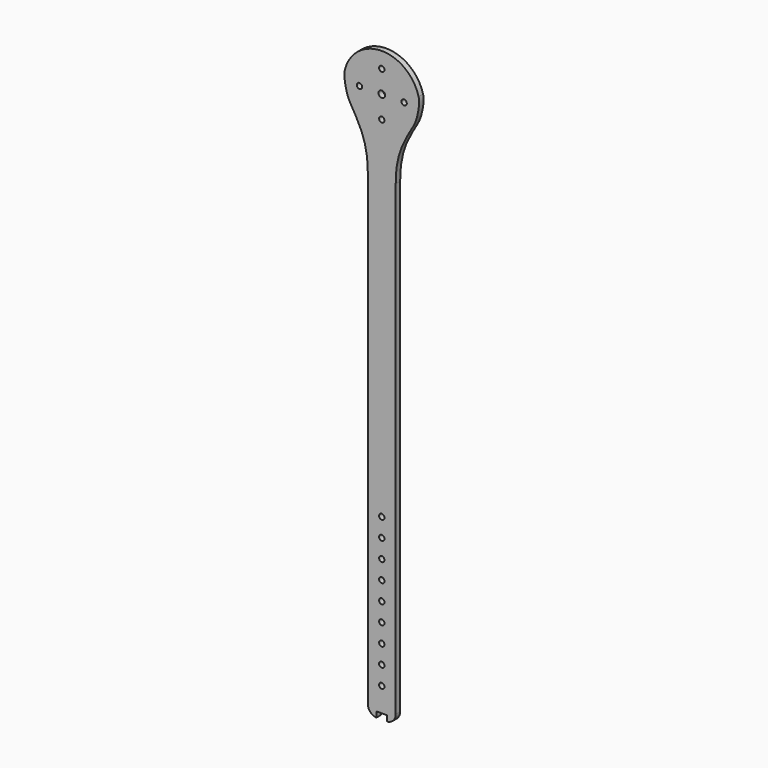
from build123d import *

# Parameters (mm, degrees)
F1_DEPTH        = 3
F2_R            = 1.7859375
F3_DEPTH        = 25
F4_T1_DEPTH     = 27.9314560345
F6_R            = 1.45
F7_DEPTH        = 25
F7_COPIES_COUNT = 4
F8_R            = 1.45
F9_DEPTH        = 25


# Not quite as in the source:
# - a fillet or chamfer that OpenCascade refuses, or shapes differently, is made with other operations: its cross-section is extruded or revolved along the edge and cut away or added
# - a pattern or mirror of a feature is missing from the dataset's text; its kind, count and spacing are read off the source's solid


with BuildPart() as f1:
    # F0 (on Front) → F1 (new body)
    with BuildSketch(Plane.XZ):
        with BuildLine():
            ThreePointArc((-17.7535207776, 10.25), (-18.9395304165, 7.8450103635), (-19.8014794389, 5.3057904246))
            add(Edge.make_bspline(
                [(-19.8014794389, 5.3057904246), (-20.454122155, 2.8700946489), (-19.9763700286, -0.7893865531), (-18.8355536126, -5.0469713795)],
                knots=[0, 0, 0, 0, 10.3977252163, 10.3977252163, 10.3977252163, 10.3977252163], degree=3))
            ThreePointArc((-18.8355536126, -5.0469713795), (-19.3331747968, 2.5452607483), (-16.8874953738, 9.75))
            Line((-16.8874953738, 9.75), (-17.7535207776, 10.25))
        make_face()
        with BuildLine():
            add(Edge.make_bspline(
                [(19.8014794389, 5.3057904246), (20.454122155, 2.8700946489), (19.9763700286, -0.7893865531), (18.8355536126, -5.0469713795)],
                knots=[0, 0, 0, 0, 10.3977252163, 10.3977252163, 10.3977252163, 10.3977252163], degree=3))
            ThreePointArc((19.8014794389, 5.3057904246), (2.6757869405, 20.3246196582), (-17.7535207776, 10.25))
            Line((-17.7535207776, 10.25), (-16.8874953738, 9.75))
            ThreePointArc((-16.8874953738, 9.75), (5.0469713795, 18.8355536126), (19.5, 0))
            ThreePointArc((19.5, 0), (19.3331747968, -2.5452607483), (18.8355536126, -5.0469713795))
        make_face()
        with BuildLine():
            ThreePointArc((-18.8355536126, -5.0469713795), (-18.015650884, -7.4623269311), (-16.8874953738, -9.75))
            ThreePointArc((-16.8874953738, -9.75), (0, -19.5), (16.8874953738, -9.75))
            ThreePointArc((16.8874953738, -9.75), (18.015650884, -7.4623269311), (18.8355536126, -5.0469713795))
            ThreePointArc((18.8355536126, -5.0469713795), (19.3331747968, -2.5452607483), (19.5, 0))
            ThreePointArc((19.5, 0), (5.0469713795, 18.8355536126), (-16.8874953738, 9.75))
            ThreePointArc((-16.8874953738, 9.75), (-19.3331747968, 2.5452607483), (-18.8355536126, -5.0469713795))
        make_face()
        with BuildLine():
            add(Edge.make_bspline(
                [(-16.8874953738, -9.75), (-15.8042909868, -11.6261650333), (-14.7498334446, -13.4051543525), (-13.7625055876, -15.1935328331)],
                knots=[0, 0, 0, 0, 6.8616960598, 6.8616960598, 6.8616960598, 6.8616960598], degree=3))
            ThreePointArc((-13.7625055876, -15.1935328331), (-0.0251276064, -20.4999846001), (13.7252177136, -15.2272255751))
            Line((13.7252177136, -15.2272255751), (14.297471583, -14.2360527984))
            add(Edge.make_bspline(
                [(16.8874953738, -9.75), (15.997662101, -11.2912364387), (15.1272281545, -12.7668954762), (14.297471583, -14.2360527984)],
                knots=[0, 0, 0, 0, 5.6367621242, 5.6367621242, 5.6367621242, 5.6367621242], degree=3))
            ThreePointArc((16.8874953738, -9.75), (0, -19.5), (-16.8874953738, -9.75))
        make_face()
        with BuildLine():
            Line((-7.5, -40), (7.5, -40))
            add(Edge.make_bspline(
                [(13.7625055876, -15.1935328331), (10.192393183, -21.6601914536), (7.5, -28.2496131611), (7.5, -40)],
                knots=[6.8616960598, 6.8616960598, 6.8616960598, 6.8616960598, 31.6731363997, 31.6731363997, 31.6731363997, 31.6731363997], degree=3))
            ThreePointArc((13.7625055876, -15.1935328331), (13.7438719752, -15.2103906304), (13.7252177136, -15.2272255751))
            ThreePointArc((13.7252177136, -15.2272255751), (-0.0251276064, -20.4999846001), (-13.7625055876, -15.1935328331))
            add(Edge.make_bspline(
                [(-13.7625055876, -15.1935328331), (-10.192393183, -21.6601914536), (-7.5, -28.2496131611), (-7.5, -40)],
                knots=[6.8616960598, 6.8616960598, 6.8616960598, 6.8616960598, 31.6731363997, 31.6731363997, 31.6731363997, 31.6731363997], degree=3))
        make_face()
        with BuildLine():
            ThreePointArc((13.7252177136, -15.2272255751), (13.7438719752, -15.2103906304), (13.7625055876, -15.1935328331))
            add(Edge.make_bspline(
                [(14.297471583, -14.2360527984), (14.1171558343, -14.5553177631), (13.9387610479, -14.8742756886), (13.7625055876, -15.1935328331)],
                knots=[5.6367621242, 5.6367621242, 5.6367621242, 5.6367621242, 6.8616960598, 6.8616960598, 6.8616960598, 6.8616960598], degree=3))
            Line((14.297471583, -14.2360527984), (13.7252177136, -15.2272255751))
        make_face()
        Polygon((7.5, -296), (7.5, -40), (-7.5, -40), (-7.5, -296), (-2.87, -296), (-2.87, -293), (2.87, -293), (2.87, -296), align=None)
    extrude(amount=F1_DEPTH)

    # F2 (on face) → F3 (cut)
    with BuildSketch(Plane.XZ.offset(3)):
        Circle(F2_R)
    extrude(amount=-F3_DEPTH, mode=Mode.SUBTRACT)

    # F4: fillet of radius 5 on 2 edges, made by hand

    # F4_s2 → F4_t1 (cut)
    with BuildSketch(Plane.XZ.offset(-12.4657280172)):
        with BuildLine():
            ThreePointArc((-7.5, -291.0137087931), (-6.1640141921, -294.4159139603), (-2.87, -296))
            Line((-2.87, -296), (-7.5, -296))
            Line((-7.5, -296), (-7.5, -291.0137087931))
        make_face()
        with BuildLine():
            ThreePointArc((7.5, -291.0137087931), (6.1640141921, -294.4159139603), (2.87, -296))
            Line((2.87, -296), (7.5, -296))
            Line((7.5, -296), (7.5, -291.0137087931))
        make_face()
    extrude(amount=F4_T1_DEPTH, mode=Mode.SUBTRACT)

    # F6 (on face) → F7 (cut)
    with BuildSketch(Plane.XZ.offset(3)):
        with Locations((0, 12)):
            Circle(F6_R)
    f7 = extrude(amount=-F7_DEPTH, mode=Mode.SUBTRACT)

    # F7_copies: F7 ×4 about axis
    f7_copies_axis = Axis((0, 0, 0), (0, 1, 0))
    for i in range(1, F7_COPIES_COUNT):
        add(f7.rotate(f7_copies_axis, i * 360 / F7_COPIES_COUNT), mode=Mode.SUBTRACT)

    # F8 (on face) → F9 (cut)
    with BuildSketch(Plane.XZ.offset(3)):
        with Locations((0, -200)):
            Circle(F8_R)
        with Locations((0, -210)):
            Circle(F8_R)
        with Locations((0, -220)):
            Circle(F8_R)
        with Locations((0, -230)):
            Circle(F8_R)
        with Locations((0, -240)):
            Circle(F8_R)
        with Locations((0, -250)):
            Circle(F8_R)
        with Locations((0, -260)):
            Circle(F8_R)
        with Locations((0, -270)):
            Circle(F8_R)
        with Locations((0, -280)):
            Circle(F8_R)
    extrude(amount=-F9_DEPTH, mode=Mode.SUBTRACT)


solid = f1.part
